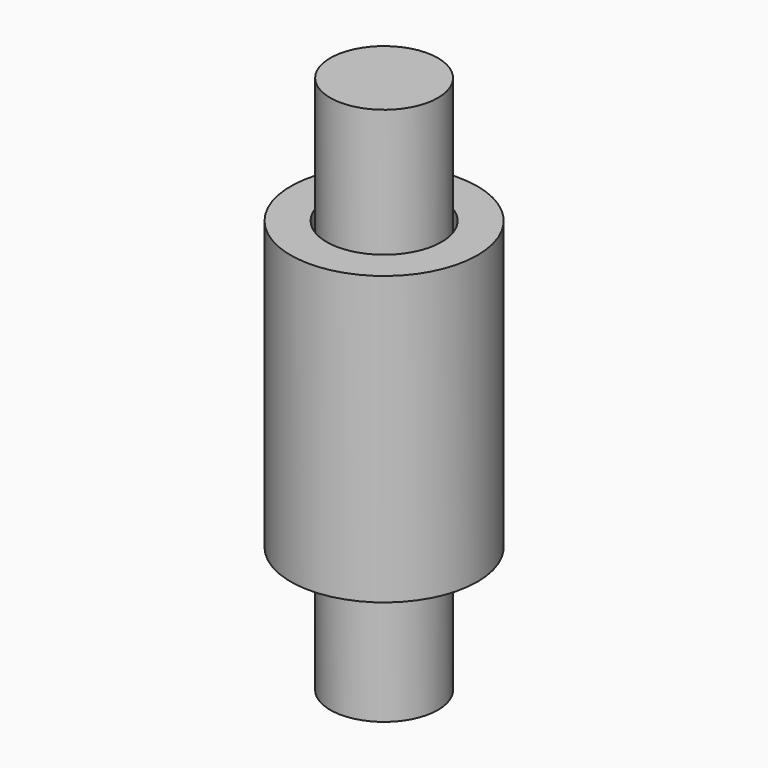
from build123d import *

# Parameters (mm, degrees)
F0_W      = 26
F0_H      = 80
F1_W      = 15
F1_H      = 35
F4_OFFSET = 1
F5_SIZE   = 4.99999
F7_DEPTH  = 25


# Not quite as in the source:
# - a fillet or chamfer is up to 0.001 mm smaller than in the source, because OpenCascade refuses the exact size
# - a feature of the source that left no trace in its solid (it failed there, or was rolled back) is left out


with BuildPart() as f2:
    # F0 (on Front) → F2 (revolve)
    with BuildSketch(Plane.XZ):
        with Locations((13, 40)):
            Rectangle(F0_W, F0_H)
    revolve(axis=Axis((0, 0, 40), (0, 0, -1)))


with BuildPart() as f3:
    # F1 (on Front) → F3 (revolve)
    with BuildSketch(Plane.XZ):
        Polygon((0, 115), (0, 0), (15, 0), (15, 10), (20, 10), (20, 70), (15, 70), (15, 115), align=None)
        with Locations((7.5, -17.5)):
            Rectangle(F1_W, F1_H)
    revolve(axis=Axis((0, 0, 40), (0, 0, -1)))


with BuildPart() as f2_1:
    add(f2.part)

    # F4: cut F3, made larger all round first
    f4_tool = offset(f3.part, amount=F4_OFFSET, kind=Kind.INTERSECTION, mode=Mode.PRIVATE)
    add(f4_tool, mode=Mode.SUBTRACT)


with BuildPart() as f3_1:
    add(f3.part)

    # F5 (size 5 in the source; OpenCascade refuses exactly that, so slightly less here)
    f5_edges = [f3_1.edges().sort_by_distance(p)[0] for p in [
        (-20, 0, 10),
    ]]
    chamfer(f5_edges, length=F5_SIZE)


with BuildPart() as f7:
    # F6 (on face) → F7 (new body)
    with BuildSketch(Plane.XY.offset(115)):
        with BuildLine():
            ThreePointArc((15, 0), (0, -15), (-15, 0))
            Line((-15, 0), (-28.4320339561, 0))
            Line((-28.4320339561, 0), (-35, -125.1360130745))
            Line((-35, -125.1360130745), (-35, -130))
            Line((-35, -130), (-10, -130))
            Line((-10, -130), (-10, -120))
            Line((-10, -120), (10, -120))
            Line((10, -120), (10, -130))
            Line((10, -130), (35, -130))
            Line((35, -130), (35, -125.1360130745))
            Line((35, -125.1360130745), (28.4320339561, 0))
            Line((28.4320339561, 0), (15, 0))
        make_face()
        with BuildLine():
            Line((15, 0), (0, 0))
            Line((0, 0), (-15, 0))
            ThreePointArc((-15, 0), (0, -15), (15, 0))
        make_face()
    extrude(amount=-F7_DEPTH)


solid = Compound([f2_1.part, f3_1.part])
